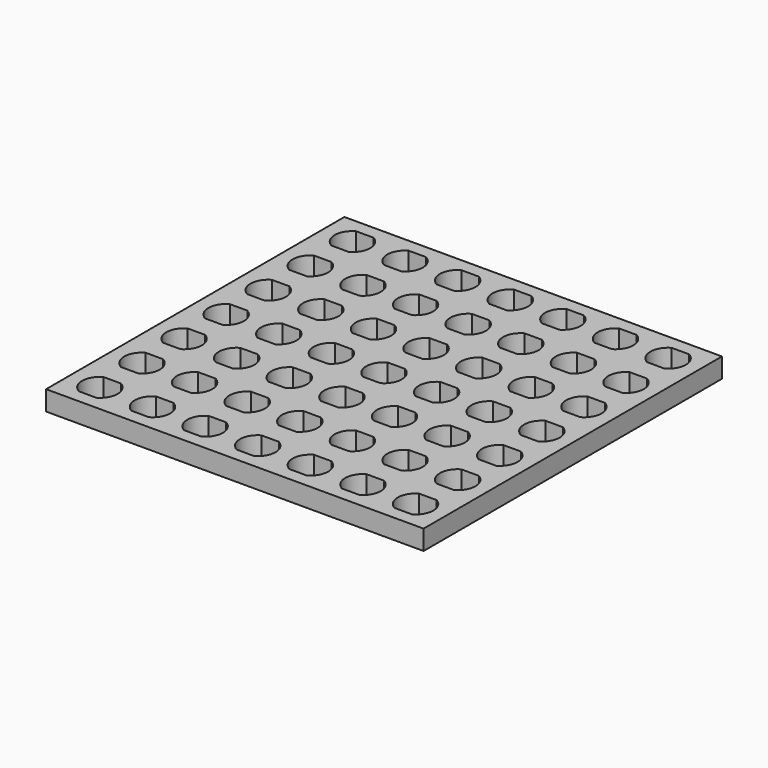
from build123d import *

# Parameters (mm, degrees)
F0_W     = 57.4
F0_H     = 56.7
F1_DEPTH = 3


# Not quite as in the source:
# - a feature of the source that left no trace in its solid (it failed there, or was rolled back) is left out


with BuildPart() as f1:
    # F0 (on Top) → F1 (new body)
    with BuildSketch(Plane.XY):
        with Locations((-0.6235789355, -7.4774807013)):
            Rectangle(F0_W, F0_H)
        with BuildLine():
            ThreePointArc((-25.9530525155, -33.8274807013), (-27.3235789355, -31.4774807013), (-25.9530525155, -29.1274807013))
            Line((-25.9530525155, -29.1274807013), (-23.2941053555, -29.1274807013))
            ThreePointArc((-23.2941053555, -29.1274807013), (-21.9235789355, -31.4774807013), (-23.2941053555, -33.8274807013))
            Line((-23.2941053555, -33.8274807013), (-25.9530525155, -33.8274807013))
        make_face(mode=Mode.SUBTRACT)
        with BuildLine():
            ThreePointArc((-17.9530525155, -33.8274807013), (-19.3235789355, -31.4774807013), (-17.9530525155, -29.1274807013))
            Line((-17.9530525155, -29.1274807013), (-15.2941053555, -29.1274807013))
            ThreePointArc((-15.2941053555, -29.1274807013), (-13.9235789355, -31.4774807013), (-15.2941053555, -33.8274807013))
            Line((-15.2941053555, -33.8274807013), (-17.9530525155, -33.8274807013))
        make_face(mode=Mode.SUBTRACT)
        with BuildLine():
            ThreePointArc((-25.9530525155, -25.8274807013), (-27.3235789355, -23.4774807013), (-25.9530525155, -21.1274807013))
            Line((-25.9530525155, -21.1274807013), (-23.2941053555, -21.1274807013))
            ThreePointArc((-23.2941053555, -21.1274807013), (-21.9235789355, -23.4774807013), (-23.2941053555, -25.8274807013))
            Line((-23.2941053555, -25.8274807013), (-25.9530525155, -25.8274807013))
        make_face(mode=Mode.SUBTRACT)
        with BuildLine():
            ThreePointArc((-17.9530525155, -25.8274807013), (-19.3235789355, -23.4774807013), (-17.9530525155, -21.1274807013))
            Line((-17.9530525155, -21.1274807013), (-15.2941053555, -21.1274807013))
            ThreePointArc((-15.2941053555, -21.1274807013), (-13.9235789355, -23.4774807013), (-15.2941053555, -25.8274807013))
            Line((-15.2941053555, -25.8274807013), (-17.9530525155, -25.8274807013))
        make_face(mode=Mode.SUBTRACT)
        with BuildLine():
            ThreePointArc((-9.9530525155, -33.8274807013), (-11.3235789355, -31.4774807013), (-9.9530525155, -29.1274807013))
            Line((-9.9530525155, -29.1274807013), (-7.2941053555, -29.1274807013))
            ThreePointArc((-7.2941053555, -29.1274807013), (-5.9235789355, -31.4774807013), (-7.2941053555, -33.8274807013))
            Line((-7.2941053555, -33.8274807013), (-9.9530525155, -33.8274807013))
        make_face(mode=Mode.SUBTRACT)
        with BuildLine():
            ThreePointArc((-9.9530525155, -25.8274807013), (-11.3235789355, -23.4774807013), (-9.9530525155, -21.1274807013))
            Line((-9.9530525155, -21.1274807013), (-7.2941053555, -21.1274807013))
            ThreePointArc((-7.2941053555, -21.1274807013), (-5.9235789355, -23.4774807013), (-7.2941053555, -25.8274807013))
            Line((-7.2941053555, -25.8274807013), (-9.9530525155, -25.8274807013))
        make_face(mode=Mode.SUBTRACT)
        with BuildLine():
            ThreePointArc((-25.9530525155, -17.8274807013), (-27.3235789355, -15.4774807013), (-25.9530525155, -13.1274807013))
            Line((-25.9530525155, -13.1274807013), (-23.2941053555, -13.1274807013))
            ThreePointArc((-23.2941053555, -13.1274807013), (-21.9235789355, -15.4774807013), (-23.2941053555, -17.8274807013))
            Line((-23.2941053555, -17.8274807013), (-25.9530525155, -17.8274807013))
        make_face(mode=Mode.SUBTRACT)
        with BuildLine():
            ThreePointArc((-17.9530525155, -17.8274807013), (-19.3235789355, -15.4774807013), (-17.9530525155, -13.1274807013))
            Line((-17.9530525155, -13.1274807013), (-15.2941053555, -13.1274807013))
            ThreePointArc((-15.2941053555, -13.1274807013), (-13.9235789355, -15.4774807013), (-15.2941053555, -17.8274807013))
            Line((-15.2941053555, -17.8274807013), (-17.9530525155, -17.8274807013))
        make_face(mode=Mode.SUBTRACT)
        with BuildLine():
            ThreePointArc((-25.9530525155, -9.8274807013), (-27.3235789355, -7.4774807013), (-25.9530525155, -5.1274807013))
            Line((-25.9530525155, -5.1274807013), (-23.2941053555, -5.1274807013))
            ThreePointArc((-23.2941053555, -5.1274807013), (-21.9235789355, -7.4774807013), (-23.2941053555, -9.8274807013))
            Line((-23.2941053555, -9.8274807013), (-25.9530525155, -9.8274807013))
        make_face(mode=Mode.SUBTRACT)
        with BuildLine():
            ThreePointArc((-17.9530525155, -9.8274807013), (-19.3235789355, -7.4774807013), (-17.9530525155, -5.1274807013))
            Line((-17.9530525155, -5.1274807013), (-15.2941053555, -5.1274807013))
            ThreePointArc((-15.2941053555, -5.1274807013), (-13.9235789355, -7.4774807013), (-15.2941053555, -9.8274807013))
            Line((-15.2941053555, -9.8274807013), (-17.9530525155, -9.8274807013))
        make_face(mode=Mode.SUBTRACT)
        with BuildLine():
            ThreePointArc((-9.9530525155, -17.8274807013), (-11.3235789355, -15.4774807013), (-9.9530525155, -13.1274807013))
            Line((-9.9530525155, -13.1274807013), (-7.2941053555, -13.1274807013))
            ThreePointArc((-7.2941053555, -13.1274807013), (-5.9235789355, -15.4774807013), (-7.2941053555, -17.8274807013))
            Line((-7.2941053555, -17.8274807013), (-9.9530525155, -17.8274807013))
        make_face(mode=Mode.SUBTRACT)
        with BuildLine():
            ThreePointArc((-9.9530525155, -9.8274807013), (-11.3235789355, -7.4774807013), (-9.9530525155, -5.1274807013))
            Line((-9.9530525155, -5.1274807013), (-7.2941053555, -5.1274807013))
            ThreePointArc((-7.2941053555, -5.1274807013), (-5.9235789355, -7.4774807013), (-7.2941053555, -9.8274807013))
            Line((-7.2941053555, -9.8274807013), (-9.9530525155, -9.8274807013))
        make_face(mode=Mode.SUBTRACT)
        with BuildLine():
            ThreePointArc((-1.9530525155, -33.8274807013), (-3.3235789355, -31.4774807013), (-1.9530525155, -29.1274807013))
            Line((-1.9530525155, -29.1274807013), (0.7058946445, -29.1274807013))
            ThreePointArc((0.7058946445, -29.1274807013), (2.0764210645, -31.4774807013), (0.7058946445, -33.8274807013))
            Line((0.7058946445, -33.8274807013), (-1.9530525155, -33.8274807013))
        make_face(mode=Mode.SUBTRACT)
        with BuildLine():
            ThreePointArc((6.0469474845, -33.8274807013), (4.6764210645, -31.4774807013), (6.0469474845, -29.1274807013))
            Line((6.0469474845, -29.1274807013), (8.7058946445, -29.1274807013))
            ThreePointArc((8.7058946445, -29.1274807013), (10.0764210645, -31.4774807013), (8.7058946445, -33.8274807013))
            Line((8.7058946445, -33.8274807013), (6.0469474845, -33.8274807013))
        make_face(mode=Mode.SUBTRACT)
        with BuildLine():
            ThreePointArc((-1.9530525155, -25.8274807013), (-3.3235789355, -23.4774807013), (-1.9530525155, -21.1274807013))
            Line((-1.9530525155, -21.1274807013), (0.7058946445, -21.1274807013))
            ThreePointArc((0.7058946445, -21.1274807013), (2.0764210645, -23.4774807013), (0.7058946445, -25.8274807013))
            Line((0.7058946445, -25.8274807013), (-1.9530525155, -25.8274807013))
        make_face(mode=Mode.SUBTRACT)
        with BuildLine():
            ThreePointArc((6.0469474845, -25.8274807013), (4.6764210645, -23.4774807013), (6.0469474845, -21.1274807013))
            Line((6.0469474845, -21.1274807013), (8.7058946445, -21.1274807013))
            ThreePointArc((8.7058946445, -21.1274807013), (10.0764210645, -23.4774807013), (8.7058946445, -25.8274807013))
            Line((8.7058946445, -25.8274807013), (6.0469474845, -25.8274807013))
        make_face(mode=Mode.SUBTRACT)
        with BuildLine():
            ThreePointArc((14.0469474845, -33.8274807013), (12.6764210645, -31.4774807013), (14.0469474845, -29.1274807013))
            Line((14.0469474845, -29.1274807013), (16.7058946445, -29.1274807013))
            ThreePointArc((16.7058946445, -29.1274807013), (18.0764210645, -31.4774807013), (16.7058946445, -33.8274807013))
            Line((16.7058946445, -33.8274807013), (14.0469474845, -33.8274807013))
        make_face(mode=Mode.SUBTRACT)
        with BuildLine():
            ThreePointArc((22.0469474845, -33.8274807013), (20.6764210645, -31.4774807013), (22.0469474845, -29.1274807013))
            Line((22.0469474845, -29.1274807013), (24.7058946445, -29.1274807013))
            ThreePointArc((24.7058946445, -29.1274807013), (26.0764210645, -31.4774807013), (24.7058946445, -33.8274807013))
            Line((24.7058946445, -33.8274807013), (22.0469474845, -33.8274807013))
        make_face(mode=Mode.SUBTRACT)
        with BuildLine():
            ThreePointArc((14.0469474845, -25.8274807013), (12.6764210645, -23.4774807013), (14.0469474845, -21.1274807013))
            Line((14.0469474845, -21.1274807013), (16.7058946445, -21.1274807013))
            ThreePointArc((16.7058946445, -21.1274807013), (18.0764210645, -23.4774807013), (16.7058946445, -25.8274807013))
            Line((16.7058946445, -25.8274807013), (14.0469474845, -25.8274807013))
        make_face(mode=Mode.SUBTRACT)
        with BuildLine():
            ThreePointArc((22.0469474845, -25.8274807013), (20.6764210645, -23.4774807013), (22.0469474845, -21.1274807013))
            Line((22.0469474845, -21.1274807013), (24.7058946445, -21.1274807013))
            ThreePointArc((24.7058946445, -21.1274807013), (26.0764210645, -23.4774807013), (24.7058946445, -25.8274807013))
            Line((24.7058946445, -25.8274807013), (22.0469474845, -25.8274807013))
        make_face(mode=Mode.SUBTRACT)
        with BuildLine():
            ThreePointArc((-1.9530525155, -17.8274807013), (-3.3235789355, -15.4774807013), (-1.9530525155, -13.1274807013))
            Line((-1.9530525155, -13.1274807013), (0.7058946445, -13.1274807013))
            ThreePointArc((0.7058946445, -13.1274807013), (2.0764210645, -15.4774807013), (0.7058946445, -17.8274807013))
            Line((0.7058946445, -17.8274807013), (-1.9530525155, -17.8274807013))
        make_face(mode=Mode.SUBTRACT)
        with BuildLine():
            ThreePointArc((6.0469474845, -17.8274807013), (4.6764210645, -15.4774807013), (6.0469474845, -13.1274807013))
            Line((6.0469474845, -13.1274807013), (8.7058946445, -13.1274807013))
            ThreePointArc((8.7058946445, -13.1274807013), (10.0764210645, -15.4774807013), (8.7058946445, -17.8274807013))
            Line((8.7058946445, -17.8274807013), (6.0469474845, -17.8274807013))
        make_face(mode=Mode.SUBTRACT)
        with BuildLine():
            ThreePointArc((-1.9530525155, -9.8274807013), (-3.3235789355, -7.4774807013), (-1.9530525155, -5.1274807013))
            Line((-1.9530525155, -5.1274807013), (0.7058946445, -5.1274807013))
            ThreePointArc((0.7058946445, -5.1274807013), (2.0764210645, -7.4774807013), (0.7058946445, -9.8274807013))
            Line((0.7058946445, -9.8274807013), (-1.9530525155, -9.8274807013))
        make_face(mode=Mode.SUBTRACT)
        with BuildLine():
            ThreePointArc((6.0469474845, -9.8274807013), (4.6764210645, -7.4774807013), (6.0469474845, -5.1274807013))
            Line((6.0469474845, -5.1274807013), (8.7058946445, -5.1274807013))
            ThreePointArc((8.7058946445, -5.1274807013), (10.0764210645, -7.4774807013), (8.7058946445, -9.8274807013))
            Line((8.7058946445, -9.8274807013), (6.0469474845, -9.8274807013))
        make_face(mode=Mode.SUBTRACT)
        with BuildLine():
            ThreePointArc((14.0469474845, -17.8274807013), (12.6764210645, -15.4774807013), (14.0469474845, -13.1274807013))
            Line((14.0469474845, -13.1274807013), (16.7058946445, -13.1274807013))
            ThreePointArc((16.7058946445, -13.1274807013), (18.0764210645, -15.4774807013), (16.7058946445, -17.8274807013))
            Line((16.7058946445, -17.8274807013), (14.0469474845, -17.8274807013))
        make_face(mode=Mode.SUBTRACT)
        with BuildLine():
            ThreePointArc((22.0469474845, -17.8274807013), (20.6764210645, -15.4774807013), (22.0469474845, -13.1274807013))
            Line((22.0469474845, -13.1274807013), (24.7058946445, -13.1274807013))
            ThreePointArc((24.7058946445, -13.1274807013), (26.0764210645, -15.4774807013), (24.7058946445, -17.8274807013))
            Line((24.7058946445, -17.8274807013), (22.0469474845, -17.8274807013))
        make_face(mode=Mode.SUBTRACT)
        with BuildLine():
            ThreePointArc((14.0469474845, -9.8274807013), (12.6764210645, -7.4774807013), (14.0469474845, -5.1274807013))
            Line((14.0469474845, -5.1274807013), (16.7058946445, -5.1274807013))
            ThreePointArc((16.7058946445, -5.1274807013), (18.0764210645, -7.4774807013), (16.7058946445, -9.8274807013))
            Line((16.7058946445, -9.8274807013), (14.0469474845, -9.8274807013))
        make_face(mode=Mode.SUBTRACT)
        with BuildLine():
            ThreePointArc((22.0469474845, -9.8274807013), (20.6764210645, -7.4774807013), (22.0469474845, -5.1274807013))
            Line((22.0469474845, -5.1274807013), (24.7058946445, -5.1274807013))
            ThreePointArc((24.7058946445, -5.1274807013), (26.0764210645, -7.4774807013), (24.7058946445, -9.8274807013))
            Line((24.7058946445, -9.8274807013), (22.0469474845, -9.8274807013))
        make_face(mode=Mode.SUBTRACT)
        with BuildLine():
            ThreePointArc((-25.9530525155, -1.8274807013), (-27.3235789355, 0.5225192987), (-25.9530525155, 2.8725192987))
            Line((-25.9530525155, 2.8725192987), (-23.2941053555, 2.8725192987))
            ThreePointArc((-23.2941053555, 2.8725192987), (-21.9235789355, 0.5225192987), (-23.2941053555, -1.8274807013))
            Line((-23.2941053555, -1.8274807013), (-25.9530525155, -1.8274807013))
        make_face(mode=Mode.SUBTRACT)
        with BuildLine():
            ThreePointArc((-17.9530525155, -1.8274807013), (-19.3235789355, 0.5225192987), (-17.9530525155, 2.8725192987))
            Line((-17.9530525155, 2.8725192987), (-15.2941053555, 2.8725192987))
            ThreePointArc((-15.2941053555, 2.8725192987), (-13.9235789355, 0.5225192987), (-15.2941053555, -1.8274807013))
            Line((-15.2941053555, -1.8274807013), (-17.9530525155, -1.8274807013))
        make_face(mode=Mode.SUBTRACT)
        with BuildLine():
            ThreePointArc((-9.9530525155, -1.8274807013), (-11.3235789355, 0.5225192987), (-9.9530525155, 2.8725192987))
            Line((-9.9530525155, 2.8725192987), (-7.2941053555, 2.8725192987))
            ThreePointArc((-7.2941053555, 2.8725192987), (-5.9235789355, 0.5225192987), (-7.2941053555, -1.8274807013))
            Line((-7.2941053555, -1.8274807013), (-9.9530525155, -1.8274807013))
        make_face(mode=Mode.SUBTRACT)
        with BuildLine():
            ThreePointArc((-25.9530525155, 6.1725192987), (-27.3235789355, 8.5225192987), (-25.9530525155, 10.8725192987))
            Line((-25.9530525155, 10.8725192987), (-23.2941053555, 10.8725192987))
            ThreePointArc((-23.2941053555, 10.8725192987), (-21.9235789355, 8.5225192987), (-23.2941053555, 6.1725192987))
            Line((-23.2941053555, 6.1725192987), (-25.9530525155, 6.1725192987))
        make_face(mode=Mode.SUBTRACT)
        with BuildLine():
            ThreePointArc((-17.9530525155, 6.1725192987), (-19.3235789355, 8.5225192987), (-17.9530525155, 10.8725192987))
            Line((-17.9530525155, 10.8725192987), (-15.2941053555, 10.8725192987))
            ThreePointArc((-15.2941053555, 10.8725192987), (-13.9235789355, 8.5225192987), (-15.2941053555, 6.1725192987))
            Line((-15.2941053555, 6.1725192987), (-17.9530525155, 6.1725192987))
        make_face(mode=Mode.SUBTRACT)
        with BuildLine():
            ThreePointArc((-23.2941053555, 18.8725192987), (-21.9235789355, 16.5225192987), (-23.2941053555, 14.1725192987))
            Line((-23.2941053555, 14.1725192987), (-25.9530525155, 14.1725192987))
            ThreePointArc((-25.9530525155, 14.1725192987), (-27.3235789355, 16.5225192987), (-25.9530525155, 18.8725192987))
            Line((-25.9530525155, 18.8725192987), (-23.2941053555, 18.8725192987))
        make_face(mode=Mode.SUBTRACT)
        with BuildLine():
            ThreePointArc((-17.9530525155, 14.1725192987), (-19.3235789355, 16.5225192987), (-17.9530525155, 18.8725192987))
            Line((-17.9530525155, 18.8725192987), (-15.2941053555, 18.8725192987))
            ThreePointArc((-15.2941053555, 18.8725192987), (-13.9235789355, 16.5225192987), (-15.2941053555, 14.1725192987))
            Line((-15.2941053555, 14.1725192987), (-17.9530525155, 14.1725192987))
        make_face(mode=Mode.SUBTRACT)
        with BuildLine():
            ThreePointArc((-9.9530525155, 6.1725192987), (-11.3235789355, 8.5225192987), (-9.9530525155, 10.8725192987))
            Line((-9.9530525155, 10.8725192987), (-7.2941053555, 10.8725192987))
            ThreePointArc((-7.2941053555, 10.8725192987), (-5.9235789355, 8.5225192987), (-7.2941053555, 6.1725192987))
            Line((-7.2941053555, 6.1725192987), (-9.9530525155, 6.1725192987))
        make_face(mode=Mode.SUBTRACT)
        with BuildLine():
            ThreePointArc((-9.9530525155, 14.1725192987), (-11.3235789355, 16.5225192987), (-9.9530525155, 18.8725192987))
            Line((-9.9530525155, 18.8725192987), (-7.2941053555, 18.8725192987))
            ThreePointArc((-7.2941053555, 18.8725192987), (-5.9235789355, 16.5225192987), (-7.2941053555, 14.1725192987))
            Line((-7.2941053555, 14.1725192987), (-9.9530525155, 14.1725192987))
        make_face(mode=Mode.SUBTRACT)
        with BuildLine():
            ThreePointArc((-1.9530525155, -1.8274807013), (-3.3235789355, 0.5225192987), (-1.9530525155, 2.8725192987))
            Line((-1.9530525155, 2.8725192987), (0.7058946445, 2.8725192987))
            ThreePointArc((0.7058946445, 2.8725192987), (2.0764210645, 0.5225192987), (0.7058946445, -1.8274807013))
            Line((0.7058946445, -1.8274807013), (-1.9530525155, -1.8274807013))
        make_face(mode=Mode.SUBTRACT)
        with BuildLine():
            ThreePointArc((6.0469474845, -1.8274807013), (4.6764210645, 0.5225192987), (6.0469474845, 2.8725192987))
            Line((6.0469474845, 2.8725192987), (8.7058946445, 2.8725192987))
            ThreePointArc((8.7058946445, 2.8725192987), (10.0764210645, 0.5225192987), (8.7058946445, -1.8274807013))
            Line((8.7058946445, -1.8274807013), (6.0469474845, -1.8274807013))
        make_face(mode=Mode.SUBTRACT)
        with BuildLine():
            ThreePointArc((14.0469474845, -1.8274807013), (12.6764210645, 0.5225192987), (14.0469474845, 2.8725192987))
            Line((14.0469474845, 2.8725192987), (16.7058946445, 2.8725192987))
            ThreePointArc((16.7058946445, 2.8725192987), (18.0764210645, 0.5225192987), (16.7058946445, -1.8274807013))
            Line((16.7058946445, -1.8274807013), (14.0469474845, -1.8274807013))
        make_face(mode=Mode.SUBTRACT)
        with BuildLine():
            ThreePointArc((22.0469474845, -1.8274807013), (20.6764210645, 0.5225192987), (22.0469474845, 2.8725192987))
            Line((22.0469474845, 2.8725192987), (24.7058946445, 2.8725192987))
            ThreePointArc((24.7058946445, 2.8725192987), (26.0764210645, 0.5225192987), (24.7058946445, -1.8274807013))
            Line((24.7058946445, -1.8274807013), (22.0469474845, -1.8274807013))
        make_face(mode=Mode.SUBTRACT)
        with BuildLine():
            ThreePointArc((-1.9530525155, 6.1725192987), (-3.3235789355, 8.5225192987), (-1.9530525155, 10.8725192987))
            Line((-1.9530525155, 10.8725192987), (0.7058946445, 10.8725192987))
            ThreePointArc((0.7058946445, 10.8725192987), (2.0764210645, 8.5225192987), (0.7058946445, 6.1725192987))
            Line((0.7058946445, 6.1725192987), (-1.9530525155, 6.1725192987))
        make_face(mode=Mode.SUBTRACT)
        with BuildLine():
            ThreePointArc((6.0469474845, 6.1725192987), (4.6764210645, 8.5225192987), (6.0469474845, 10.8725192987))
            Line((6.0469474845, 10.8725192987), (8.7058946445, 10.8725192987))
            ThreePointArc((8.7058946445, 10.8725192987), (10.0764210645, 8.5225192987), (8.7058946445, 6.1725192987))
            Line((8.7058946445, 6.1725192987), (6.0469474845, 6.1725192987))
        make_face(mode=Mode.SUBTRACT)
        with BuildLine():
            ThreePointArc((-1.9530525155, 14.1725192987), (-3.3235789355, 16.5225192987), (-1.9530525155, 18.8725192987))
            Line((-1.9530525155, 18.8725192987), (0.7058946445, 18.8725192987))
            ThreePointArc((0.7058946445, 18.8725192987), (2.0764210645, 16.5225192987), (0.7058946445, 14.1725192987))
            Line((0.7058946445, 14.1725192987), (-1.9530525155, 14.1725192987))
        make_face(mode=Mode.SUBTRACT)
        with BuildLine():
            ThreePointArc((6.0469474845, 14.1725192987), (4.6764210645, 16.5225192987), (6.0469474845, 18.8725192987))
            Line((6.0469474845, 18.8725192987), (8.7058946445, 18.8725192987))
            ThreePointArc((8.7058946445, 18.8725192987), (10.0764210645, 16.5225192987), (8.7058946445, 14.1725192987))
            Line((8.7058946445, 14.1725192987), (6.0469474845, 14.1725192987))
        make_face(mode=Mode.SUBTRACT)
        with BuildLine():
            ThreePointArc((14.0469474845, 6.1725192987), (12.6764210645, 8.5225192987), (14.0469474845, 10.8725192987))
            Line((14.0469474845, 10.8725192987), (16.7058946445, 10.8725192987))
            ThreePointArc((16.7058946445, 10.8725192987), (18.0764210645, 8.5225192987), (16.7058946445, 6.1725192987))
            Line((16.7058946445, 6.1725192987), (14.0469474845, 6.1725192987))
        make_face(mode=Mode.SUBTRACT)
        with BuildLine():
            ThreePointArc((22.0469474845, 6.1725192987), (20.6764210645, 8.5225192987), (22.0469474845, 10.8725192987))
            Line((22.0469474845, 10.8725192987), (24.7058946445, 10.8725192987))
            ThreePointArc((24.7058946445, 10.8725192987), (26.0764210645, 8.5225192987), (24.7058946445, 6.1725192987))
            Line((24.7058946445, 6.1725192987), (22.0469474845, 6.1725192987))
        make_face(mode=Mode.SUBTRACT)
        with BuildLine():
            ThreePointArc((14.0469474845, 14.1725192987), (12.6764210645, 16.5225192987), (14.0469474845, 18.8725192987))
            Line((14.0469474845, 18.8725192987), (16.7058946445, 18.8725192987))
            ThreePointArc((16.7058946445, 18.8725192987), (18.0764210645, 16.5225192987), (16.7058946445, 14.1725192987))
            Line((16.7058946445, 14.1725192987), (14.0469474845, 14.1725192987))
        make_face(mode=Mode.SUBTRACT)
        with BuildLine():
            ThreePointArc((22.0469474845, 14.1725192987), (20.6764210645, 16.5225192987), (22.0469474845, 18.8725192987))
            Line((22.0469474845, 18.8725192987), (24.7058946445, 18.8725192987))
            ThreePointArc((24.7058946445, 18.8725192987), (26.0764210645, 16.5225192987), (24.7058946445, 14.1725192987))
            Line((24.7058946445, 14.1725192987), (22.0469474845, 14.1725192987))
        make_face(mode=Mode.SUBTRACT)
    extrude(amount=F1_DEPTH)


solid = f1.part
